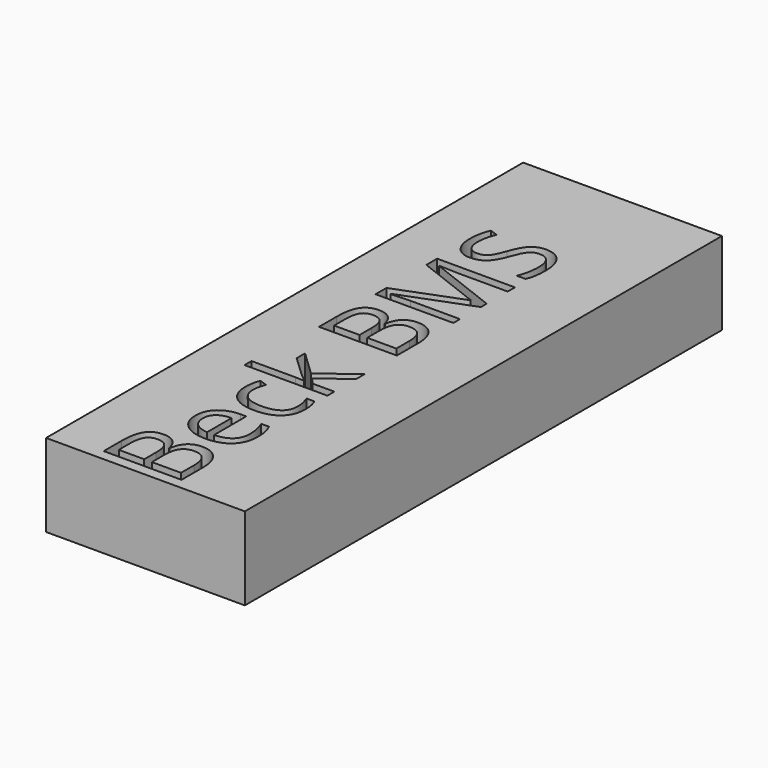
from build123d import *

# Parameters (mm, degrees)
F0_W         = 76.2
F0_H         = 228.6
F1_DEPTH     = 31.75
F2_TEXT_SIZE = 41.7768229172
F3_DEPTH     = 25.4


# Not quite as in the source:
# - Text() gives the source's letters only with a copy of the font that has no kerning and outlines rounded to 1/6400 em; it was checked with that copy


with BuildPart() as f1:
    # F0 (on Top) → F1 (new body)
    with BuildSketch(Plane.XY):
        with Locations((38.1, 114.3)):
            Rectangle(F0_W, F0_H)
    extrude(amount=F1_DEPTH)

    # F2 (on face) → F3 (cut)
    with BuildSketch(Plane.XY.offset(31.75)):
        with Locations(Location((48.631651438, 0), (0, 0, 90))):
            Text('Beck BMS', F2_TEXT_SIZE, font='Open Sans', text_align=(TextAlign.LEFT, TextAlign.BOTTOM))
    extrude(amount=-F3_DEPTH, mode=Mode.SUBTRACT)


solid = f1.part
